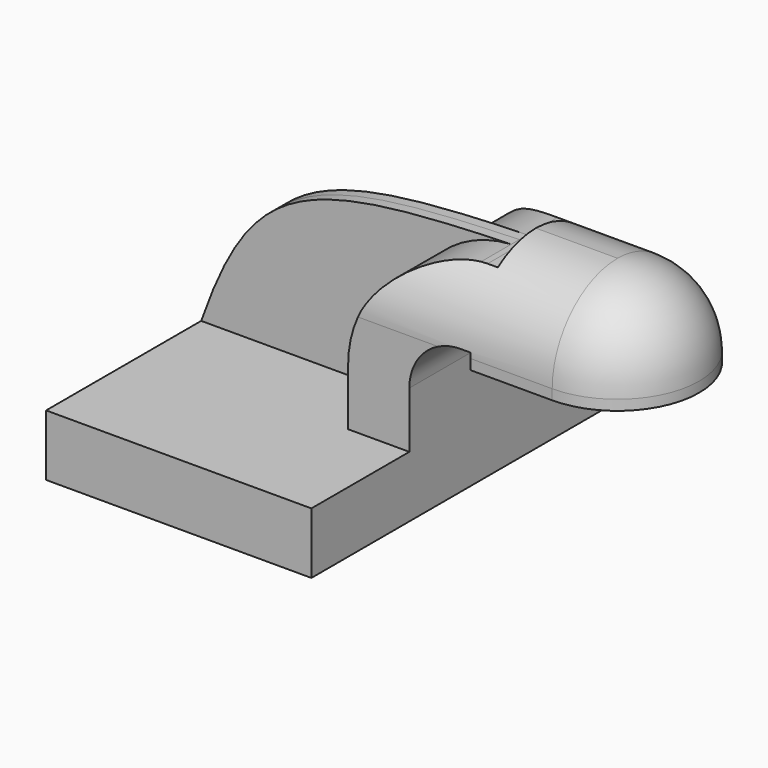
from build123d import *

# Parameters (mm, degrees)
F1_DEPTH     = 63.5
F0_W         = 25.4
F0_H         = 19.05
F0_H_2       = 4.7752
F0_H_3       = 4.7498
F2_DEPTH     = 25.4
F3_DEPTH     = 3.175
F5_T1_DEPTH  = 88.9
F5_T4_ANGLE  = 180
F6_T         = 2.54
F6_T3_DEPTH  = 24.13
F6_T5_DEPTH  = 27.305
F6_T7_DEPTH  = 68.58
F6_T9_DEPTH  = 27.305
F6_T11_DEPTH = 22.5552
F6_T13_DEPTH = 55.7790871697
F6_T15_DEPTH = 34.6589952471
F6_T18_ANGLE = 86.7817435726
F6_T20_ANGLE = 86.7817435726


# Not quite as in the source:
# - a fillet or chamfer that OpenCascade refuses, or shapes differently, is made with other operations: its cross-section is extruded or revolved along the edge and cut away or added
# - a shell that OpenCascade refuses in one call is made with other operations: the cavity is built on its own and cut out


with BuildPart() as f1:
    # F0 (on Front) → F1 (new body, symmetric)
    with BuildSketch(Plane.XZ):
        Polygon((41.275, -9.525), (41.275, 9.525), (22.225, 9.525), (-41.275, 9.525), (-41.275, -9.525), align=None)
    extrude(amount=F1_DEPTH, both=True)

    # F0 (on Front) → F2 (join, symmetric)
    with BuildSketch(Plane.XZ):
        with BuildLine():
            Line((22.225, 9.525), (41.275, 9.525))
            Line((41.275, 9.525), (41.275, 27.0002))
            ThreePointArc((41.275, 27.0002), (45.9246798487, 38.2255201513), (57.15, 42.8752))
            Line((57.15, 42.8752), (60.325, 42.8752))
            Line((60.325, 42.8752), (60.325, 61.9252))
            Line((60.325, 61.9252), (57.15, 61.9252))
            add(Edge.make_bspline(
                [(55.1893230691, 61.8701207193), (55.8379631981, 61.8888818572), (56.4915059272, 61.9072303668), (57.15, 61.9252)],
                knots=[110.4053566359, 110.4053566359, 110.4053566359, 110.4053566359, 111.5045361635, 111.5045361635, 111.5045361635, 111.5045361635], degree=3))
            ThreePointArc((55.1893230691, 61.8701207193), (31.7705568736, 50.9926882326), (22.225, 27.0002))
            Line((22.225, 27.0002), (22.225, 9.525))
        make_face()
        with Locations((73.025, 52.4002)):
            Rectangle(F0_W, F0_H)
        with Locations((73.025, 40.4876)):
            Rectangle(F0_W, F0_H_2)
        with Locations((73.025, 64.3001)):
            Rectangle(F0_W, F0_H_3)
    extrude(amount=F2_DEPTH, both=True)

    # F0 (on Front) → F3 (join, symmetric)
    with BuildSketch(Plane.XZ):
        with BuildLine():
            Line((-41.275, 9.525), (22.225, 9.525))
            Line((22.225, 9.525), (22.225, 27.0002))
            ThreePointArc((22.225, 27.0002), (31.7705568736, 50.9926882326), (55.1893230691, 61.8701207193))
            add(Edge.make_bspline(
                [(-41.275, 9.525), (-25.6521962788, 53.9382967597), (-9.9623131958, 59.9856877717), (55.1893230691, 61.8701207193)],
                knots=[0, 0, 0, 0, 110.4053566359, 110.4053566359, 110.4053566359, 110.4053566359], degree=3))
        make_face()
    extrude(amount=F3_DEPTH, both=True)

    # F0 (on Front) → F4 (revolve)
    with BuildSketch(Plane.XZ):
        Polygon((85.725, 61.9252), (85.725, 42.8752), (85.725, 38.1), (111.125, 38.1), (111.125, 66.675), (85.725, 66.675), align=None)
    revolve(axis=Axis((85.725, 0, 52.3875), (0, 0, 1)))

    # F5: fillet of radius 25.4 on 1 edges, made by hand

    # F5_s2 → F5_t1 (cut)
    with BuildSketch(Plane.YZ.offset(-3.175)):
        with BuildLine():
            ThreePointArc((0, 66.675), (17.9605122421, 59.2355122421), (25.4, 41.275))
            Line((25.4, 41.275), (25.4, 66.675))
            Line((25.4, 66.675), (0, 66.675))
        make_face()
        with BuildLine():
            ThreePointArc((0, 66.675), (-17.9605122421, 59.2355122421), (-25.4, 41.275))
            Line((-25.4, 41.275), (-25.4, 66.675))
            Line((-25.4, 66.675), (0, 66.675))
        make_face()
    extrude(amount=F5_T1_DEPTH, mode=Mode.SUBTRACT)

    # F5_s3 → F5_t4 (revolve, cut)
    with BuildSketch(Plane.YZ.offset(85.725)):
        with BuildLine():
            ThreePointArc((0, 66.675), (17.9605122421, 59.2355122421), (25.4, 41.275))
            Line((25.4, 41.275), (25.4, 66.675))
            Line((25.4, 66.675), (0, 66.675))
        make_face()
    revolve(axis=Axis((85.725, 0, 66.675), (0, 0, -1)), revolution_arc=F5_T4_ANGLE, mode=Mode.SUBTRACT)

    # F6: shell of thickness 2.54, made by hand


with BuildPart() as f6_core1:
    # F6_t2: copy of F1
    add(f1.part)

    # the walls: a layer under each face that stays
    f6_faces = [f6_core1.faces().sort_by_distance(p)[0] for p in [
        (41.275, 0, 8.7376),
        (0, 63.5, 0),
        (0, 33.3375, 9.525),
        (36.214543408, 25.4, 25.4),
        (45.9246798487, 0, 38.2255201513),
        (36.214543408, -25.4, 25.4),
        (0, -33.3375, 9.525),
        (0, -63.5, 0),
        (-41.275, 0, 0),
        (22.225, 14.2875, 18.2626),
        (6.9571615345, 3.175, 35.6975603597),
        (31.7705568736, 14.2875, 50.9926882326),
        (55.5002346295, 17.9605122421, 59.2355122421),
        (55.5002346295, -17.9605122421, 59.2355122421),
        (58.7375, 0, 42.8752),
        (31.7705568736, -14.2875, 50.9926882326),
        (22.225, -14.2875, 18.2626),
        (6.9571615345, -3.175, 35.6975603597),
        (-11.6161506693, 1.5875, 51.6458842892),
        (-11.6161506693, -1.5875, 51.6458842892),
        (56.1659663056, 7.4330512334, 61.8979571739),
        (60.325, 0, 64.3001),
        (58.7375, 0, 61.9252),
        (60.325, 0, 40.4876),
        (73.025, 25.4, 39.6875),
        (103.6855122422, -1e-10, 59.2355122421),
        (56.1659663056, -7.4330512334, 61.8979571739),
        (73.025, -25.4, 39.6875),
        (85.725, 0, 38.1),
        (111.125, 0, 39.6875),
    ]]
    thicken(f6_faces, amount=-F6_T, mode=Mode.SUBTRACT)

    # F6_s4 → F6_t3 (cut)
    with BuildSketch(Plane.YZ.offset(19.685)):
        Polygon((25.4254, 9.5504), (25.4, 6.985), (22.86, 6.985), (22.86, 9.525), align=None)
        Polygon((-25.4254, 9.5504), (-22.86, 9.525), (-22.86, 6.985), (-25.4, 6.985), align=None)
    extrude(amount=F6_T3_DEPTH, mode=Mode.SUBTRACT)

    # F6_s6 → F6_t5 (cut)
    with BuildSketch(Plane.XZ.offset(-27.94)):
        Polygon((22.1996, 9.5504), (22.225, 6.985), (24.765, 6.985), (24.765, 9.525), align=None)
    extrude(amount=F6_T5_DEPTH, mode=Mode.SUBTRACT)

    # F6_s8 → F6_t7 (cut)
    with BuildSketch(Plane.YZ.offset(-43.815)):
        Polygon((3.2004, 9.5504), (3.175, 6.985), (0.635, 6.985), (0.635, 9.525), align=None)
        Polygon((-3.2004, 9.5504), (-3.175, 6.985), (-0.635, 6.985), (-0.635, 9.525), align=None)
    extrude(amount=F6_T7_DEPTH, mode=Mode.SUBTRACT)

    # F6_s10 → F6_t9 (cut)
    with BuildSketch(Plane.XZ.offset(0.635)):
        Polygon((22.1996, 9.5504), (22.225, 6.985), (24.765, 6.985), (24.765, 9.525), align=None)
    extrude(amount=F6_T9_DEPTH, mode=Mode.SUBTRACT)

    # F6_s12 → F6_t11 (cut)
    with BuildSketch(Plane.XY.offset(6.985)):
        Polygon((22.1996, 3.2004), (24.765, 3.175), (24.765, 0.635), (22.225, 0.635), align=None)
        Polygon((22.1996, -3.2004), (24.765, -3.175), (24.765, -0.635), (22.225, -0.635), align=None)
    extrude(amount=F6_T11_DEPTH, mode=Mode.SUBTRACT)

    # F6_s14 → F6_t13 (cut)
    with BuildSketch(Plane.XZ.offset(-27.8895435848)):
        Polygon((60.2996, 42.8498), (60.325, 45.4152), (62.865, 45.4152), (62.865, 42.8752), align=None)
    extrude(amount=F6_T13_DEPTH, mode=Mode.SUBTRACT)

    # F6_s16 → F6_t15 (cut)
    with BuildSketch(Plane.XZ.offset(-17.3294976236)):
        Polygon((60.2996, 61.9506), (62.865, 61.9252), (62.865, 59.3852), (60.325, 59.3852), align=None)
    extrude(amount=F6_T15_DEPTH, mode=Mode.SUBTRACT)

    # F6_s17 → F6_t18 (revolve, cut)
    with BuildSketch(Plane.XY.offset(27.0002)):
        Polygon((22.1996, 3.2004), (22.225, 0.635), (24.765, 0.635), (24.765, 3.175), align=None)
    revolve(axis=Axis((57.15, 3.175, 27.0002), (0, 1, 0)), revolution_arc=F6_T18_ANGLE, mode=Mode.SUBTRACT)

    # F6_s19 → F6_t20 (revolve, cut)
    with BuildSketch(Plane.XY.offset(27.0002)):
        Polygon((22.1996, -3.2004), (24.765, -3.175), (24.765, -0.635), (22.225, -0.635), align=None)
    revolve(axis=Axis((57.15, -3.175, 27.0002), (0, 1, 0)), revolution_arc=F6_T20_ANGLE, mode=Mode.SUBTRACT)


with BuildPart() as f1_1:
    add(f1.part)

    # what is left inside the walls is the cavity
    f6_cavity = [f6_core1.part.solids().sort_by_distance(p)[0] for p in [
        (0, 20.32, -9.4996),
    ]]
    add(f6_cavity, mode=Mode.SUBTRACT)


solid = f1_1.part
